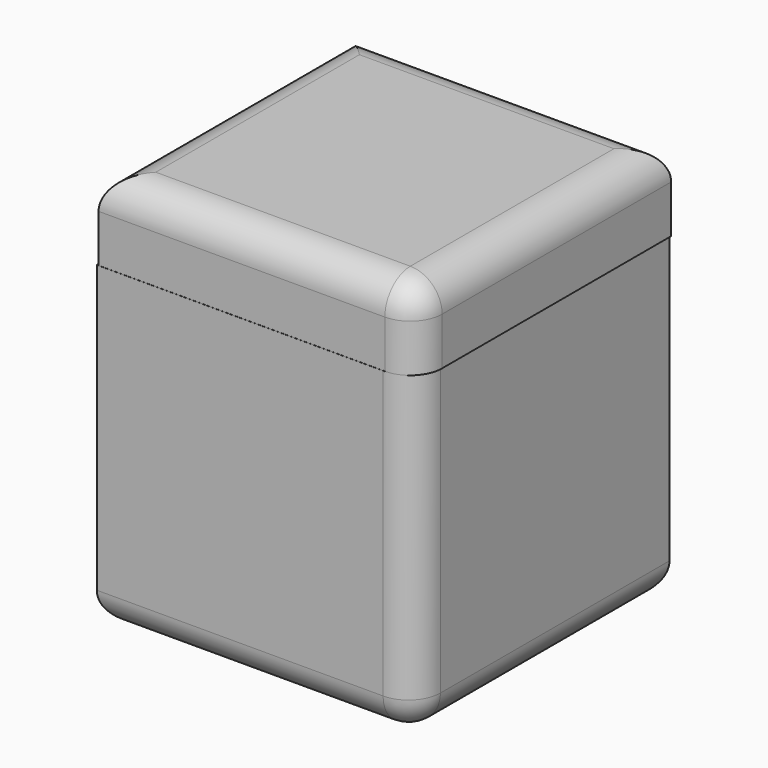
from build123d import *

# Parameters (mm, degrees)
F0_W         = 100
F0_H         = 100
F1_DEPTH     = 100
F2_T         = -10
F3_W         = 80
F3_H         = 10
F4_DEPTH     = 100
F6_W         = 100
F6_H         = 100
F7_DEPTH     = 25
F8_R         = 10
F9_R         = 10
F10_T1_DEPTH = 90
F10_S5_W     = 10
F10_S5_H     = 10
F10_T6_DEPTH = 10
F11_T1_DEPTH = 15
F11_S5_W     = 10.2
F11_S5_H     = 10.2
F11_T6_DEPTH = 10.2


# Not quite as in the source:
# - a fillet or chamfer that OpenCascade refuses, or shapes differently, is made with other operations: its cross-section is extruded or revolved along the edge and cut away or added


with BuildPart() as f1:
    # F0 (on Top) → F1 (new body)
    with BuildSketch(Plane.XY):
        Rectangle(F0_W, F0_H)
    extrude(amount=F1_DEPTH)

    # F2
    f2_openings = [f1.faces().sort_by_distance(p)[0] for p in [
        (0, 0, 100),
    ]]
    offset(amount=F2_T, openings=f2_openings)

    # F3 (on Top) → F4 (join)
    with BuildSketch(Plane.XY):
        Rectangle(F3_W, F3_H)
    extrude(amount=F4_DEPTH)

    # F6 (on offset) → F7 (join)
    with BuildSketch(Plane.XY.offset(100)):
        with Locations((0.513449031, 0.0360049307)):
            Rectangle(F6_W, F6_H)
    extrude(amount=F7_DEPTH)

    # F8
    f8_edges = [f1.edges().sort_by_distance(p)[0] for p in [
        (0.513449, 50.036005, 125),
        (-49.486551, 0.036005, 125),
        (0.513449, -49.963995, 125),
        (50.513449, 0.036005, 125),
    ]]
    fillet(f8_edges, radius=F8_R)

    # F9
    f9_edges = [f1.edges().sort_by_distance(p)[0] for p in [
        (0, -50, 0),
        (50, 0, 0),
        (0, 50, 0),
        (-50, 0, 0),
    ]]
    fillet(f9_edges, radius=F9_R)

    # F10: fillet of radius 10 on 1 edges, made by hand

    # F10_s2 → F10_t1 (cut)
    with BuildSketch(Plane.XY.offset(10)):
        with BuildLine():
            ThreePointArc((50, -40), (47.0710678119, -47.0710678119), (40, -50))
            Line((40, -50), (50, -50))
            Line((50, -50), (50, -40))
        make_face()
    extrude(amount=F10_T1_DEPTH, mode=Mode.SUBTRACT)


with BuildPart() as f10_tool4:
    # F10_s5 → F10_t6 (new body)
    with BuildSketch(Plane.YZ.offset(40)):
        with Locations((-45, 5)):
            Rectangle(F10_S5_W, F10_S5_H)
    extrude(amount=F10_T6_DEPTH)

    # F10_s7 → F10_t8 (revolve, cut)
    with BuildSketch(Plane(origin=(40, -40, 10), x_dir=(0, 0.7071067812, 0.7071067812), z_dir=(0, 0.7071067812, -0.7071067812))):
        with BuildLine():
            ThreePointArc((0, -10), (10, 0), (0, 10))
            Line((0, 10), (0, -10))
        make_face()
    revolve(axis=Axis((40, -40, 10), (1, 0, 0)), mode=Mode.SUBTRACT)


with BuildPart() as f1_1:
    add(f1.part)

    # F10_t3: cut F10_tool4
    add(f10_tool4.part, mode=Mode.SUBTRACT)

    # F11: fillet of radius 10 on 1 edges, made by hand

    # F11_s2 → F11_t1 (cut)
    with BuildSketch(Plane.XY.offset(100)):
        with BuildLine():
            ThreePointArc((50.513449031, -39.9639950693), (47.5845168429, -47.0350628811), (40.513449031, -49.9639950693))
            Line((40.513449031, -49.9639950693), (50.513449031, -49.9639950693))
            Line((50.513449031, -49.9639950693), (50.513449031, -39.9639950693))
        make_face()
    extrude(amount=F11_T1_DEPTH, mode=Mode.SUBTRACT)


with BuildPart() as f11_tool4:
    # F11_s5 → F11_t6 (new body)
    with BuildSketch(Plane.YZ.offset(40.513449031)):
        with Locations((-45.0639950693, 120.1)):
            Rectangle(F11_S5_W, F11_S5_H)
    extrude(amount=F11_T6_DEPTH)

    # F11_s7 → F11_t8 (revolve, cut)
    with BuildSketch(Plane(origin=(40.513449031, -39.9639950693, 115), x_dir=(0, 0.7071067812, -0.7071067812), z_dir=(0, -0.7071067812, -0.7071067812))):
        with BuildLine():
            ThreePointArc((0, -10), (10, 0), (0, 10))
            Line((0, 10), (0, -10))
        make_face()
    revolve(axis=Axis((40.513449031, -39.9639950693, 115), (1, 0, 0)), mode=Mode.SUBTRACT)


with BuildPart() as f1_2:
    add(f1_1.part)

    # F11_t3: cut F11_tool4
    add(f11_tool4.part, mode=Mode.SUBTRACT)


solid = f1_2.part
